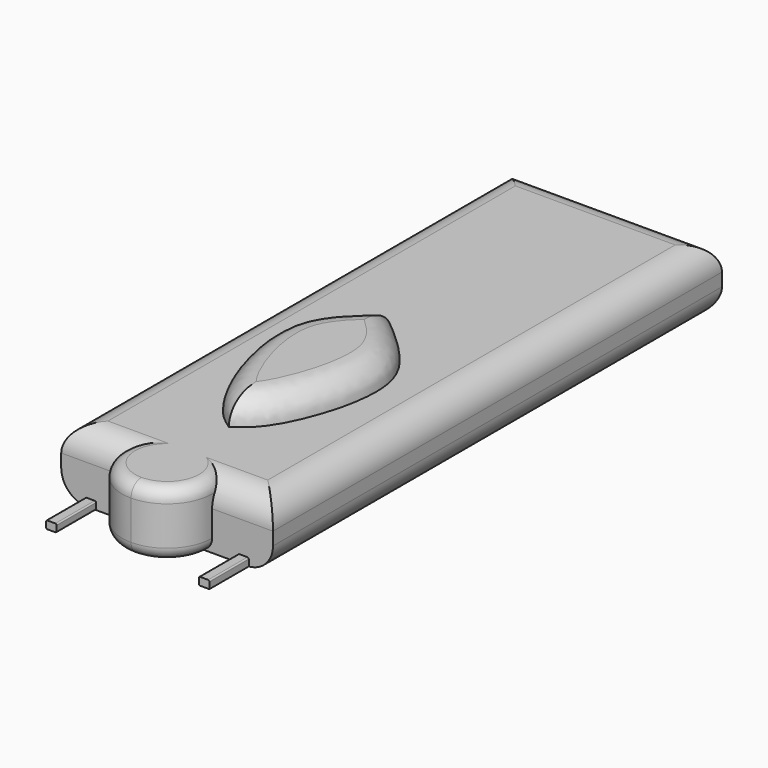
from build123d import *

# Parameters (mm, degrees)
F0_W     = 2.070606
F0_H     = 9.613432
F1_DEPTH = 12.7
F2_DEPTH = 17.78
F3_DEPTH = 12.7
F4_DEPTH = 1.524
F5_R     = 5.08
F6_R     = 2.54
F7_R     = 5.079
F8_R     = 0.254
F9_DEPTH = 12.7


# Not quite as in the source:
# - a fillet or chamfer is up to 0.001 mm smaller than in the source, because OpenCascade refuses the exact size


with BuildPart() as f1:
    # F0 (on Top) → F1 (new body)
    with BuildSketch(Plane.XY):
        with BuildLine():
            Line((0, 27.361285), (0, 54.870538))
            Line((0, 54.870538), (-20.705864, 54.870538))
            Line((-20.705864, 54.870538), (-20.705864, -54.870538))
            Line((-20.705864, -54.870538), (-15.973106, -54.870538))
            Line((-15.973106, -54.870538), (-15.973106, -45.257106))
            Line((-15.973106, -45.257106), (-13.9025, -45.257106))
            Line((-13.9025, -45.257106), (-13.9025, -54.870538))
            Line((-13.9025, -54.870538), (-8.805898, -54.870538))
            ThreePointArc((-8.805898, -54.870538), (-6.22671, -48.643828), (0, -46.06464))
            Line((0, -46.06464), (0, -39.784834))
            add(Edge.make_bspline(
                [(0, 0), (-4.492536, -3.747644), (-14.112193, -11.772303), (-6.206922, -35.481695), (-1.653336, -38.638613), (0, -39.784834)],
                knots=[0, 0, 0, 0, 0.358186, 0.766967, 1, 1, 1, 1], degree=3))
            Line((0, 0), (0, 4.556645))
            ThreePointArc((0, 4.556645), (-11.40232, 15.958965), (0, 27.361285))
        make_face()
        with BuildLine():
            Line((20.705864, -54.870538), (20.705864, 54.870538))
            Line((20.705864, 54.870538), (0, 54.870538))
            Line((0, 54.870538), (0, 27.361285))
            ThreePointArc((0, 27.361285), (8.062658, 24.021623), (11.40232, 15.958965))
            ThreePointArc((11.40232, 15.958965), (8.062658, 7.896307), (0, 4.556645))
            Line((0, 4.556645), (0, 0))
            add(Edge.make_bspline(
                [(0, 0), (4.492536, -3.747644), (14.112193, -11.772303), (6.206922, -35.481695), (1.653336, -38.638613), (0, -39.784834)],
                knots=[0, 0, 0, 0, 0.358186, 0.766967, 1, 1, 1, 1], degree=3))
            Line((0, -39.784834), (0, -46.06464))
            ThreePointArc((0, -46.06464), (6.22671, -48.643828), (8.805898, -54.870538))
            Line((8.805898, -54.870538), (13.9025, -54.870538))
            Line((13.9025, -54.870538), (13.9025, -45.257106))
            Line((13.9025, -45.257106), (15.973106, -45.257106))
            Line((15.973106, -45.257106), (15.973106, -54.870538))
            Line((15.973106, -54.870538), (20.705864, -54.870538))
        make_face()
        with Locations((14.937803, -50.063822)):
            Rectangle(F0_W, F0_H)
        with Locations((-14.937803, -50.063822)):
            Rectangle(F0_W, F0_H)
        with BuildLine():
            Line((-8.805898, -54.870538), (0, -54.870538))
            Line((0, -54.870538), (0, -46.06464))
            ThreePointArc((0, -46.06464), (-6.22671, -48.643828), (-8.805898, -54.870538))
        make_face()
        with BuildLine():
            Line((0, -54.870538), (8.805898, -54.870538))
            ThreePointArc((8.805898, -54.870538), (6.22671, -48.643828), (0, -46.06464))
            Line((0, -46.06464), (0, -54.870538))
        make_face()
    extrude(amount=F1_DEPTH)

    # F0 (on Top) → F2 (join)
    with BuildSketch(Plane.XY):
        with BuildLine():
            Line((0, -39.784834), (0, 0))
            add(Edge.make_bspline(
                [(0, 0), (-4.492536, -3.747644), (-14.112193, -11.772303), (-6.206922, -35.481695), (-1.653336, -38.638613), (0, -39.784834)],
                knots=[0, 0, 0, 0, 0.358186, 0.766967, 1, 1, 1, 1], degree=3))
        make_face()
        with BuildLine():
            add(Edge.make_bspline(
                [(0, 0), (4.492536, -3.747644), (14.112193, -11.772303), (6.206922, -35.481695), (1.653336, -38.638613), (0, -39.784834)],
                knots=[0, 0, 0, 0, 0.358186, 0.766967, 1, 1, 1, 1], degree=3))
            Line((0, 0), (0, -39.784834))
        make_face()
    extrude(amount=F2_DEPTH)

    # F0 (on Top) → F3 (join)
    with BuildSketch(Plane.XY):
        with BuildLine():
            Line((0, -63.676437), (0, -54.870538))
            Line((0, -54.870538), (-8.805898, -54.870538))
            ThreePointArc((-8.805898, -54.870538), (-6.22671, -61.097249), (0, -63.676437))
        make_face()
        with BuildLine():
            ThreePointArc((0, -63.676437), (6.22671, -61.097249), (8.805898, -54.870538))
            Line((8.805898, -54.870538), (0, -54.870538))
            Line((0, -54.870538), (0, -63.676437))
        make_face()
    extrude(amount=F3_DEPTH)

    # F0 (on Top) → F4 (join)
    with BuildSketch(Plane.XY):
        with Locations((14.937803, -59.677254)):
            Rectangle(F0_W, F0_H)
        with Locations((-14.937803, -59.677254)):
            Rectangle(F0_W, F0_H)
    extrude(amount=F4_DEPTH)

    # F5
    f5_edges = [f1.edges().sort_by_distance(p)[0] for p in [
        (-20.705864, 0, 12.7),
        (-20.705864, 0, 0),
        (0, 54.870538, 12.7),
        (0, 54.870538, 0),
        (20.705864, 0, 12.7),
        (14.755881, -54.870538, 12.7),
        (20.705864, 0, 0),
        (-14.755881, -54.870538, 12.7),
    ]]
    fillet(f5_edges, radius=F5_R)

    # F6
    f6_edges = [f1.edges().sort_by_distance(p)[0] for p in [
        (-8.39296, -52.205569, 12.7),
        (0, -63.676437, 12.7),
        (8.39296, -52.205569, 12.7),
        (0, -63.676437, 0),
    ]]
    fillet(f6_edges, radius=F6_R)

    # F7 (radius 5.08 in the source; OpenCascade refuses exactly that, so slightly less here)
    f7_edges = [f1.edges().sort_by_distance(p)[0] for p in [
        (-10.152826, -19.56667, 17.78),
        (10.152826, -19.56667, 17.78),
    ]]
    fillet(f7_edges, radius=F7_R)

    # F8
    f8_edges = [f1.edges().sort_by_distance(p)[0] for p in [
        (15.973106, -59.677254, 1.524),
        (15.625864, -7.346716, 0),
        (13.9025, -59.677254, 1.524),
        (13.9025, -59.677254, 0),
        (-15.973106, -59.677254, 1.524),
        (-15.973106, -59.677254, 0.011882),
        (-13.9025, -59.677254, 1.524),
        (-13.9025, -59.677254, 0),
    ]]
    fillet(f8_edges, radius=F8_R)

    # F0 (on Top) → F9 (join)
    with BuildSketch(Plane.XY):
        with BuildLine():
            ThreePointArc((11.40232, 15.958965), (8.062658, 24.021623), (0, 27.361285))
            Line((0, 27.361285), (0, 4.556645))
            ThreePointArc((0, 4.556645), (8.062658, 7.896307), (11.40232, 15.958965))
        make_face()
        with BuildLine():
            Line((0, 4.556645), (0, 27.361285))
            ThreePointArc((0, 27.361285), (-11.40232, 15.958965), (0, 4.556645))
        make_face()
    extrude(amount=F9_DEPTH)


solid = f1.part
